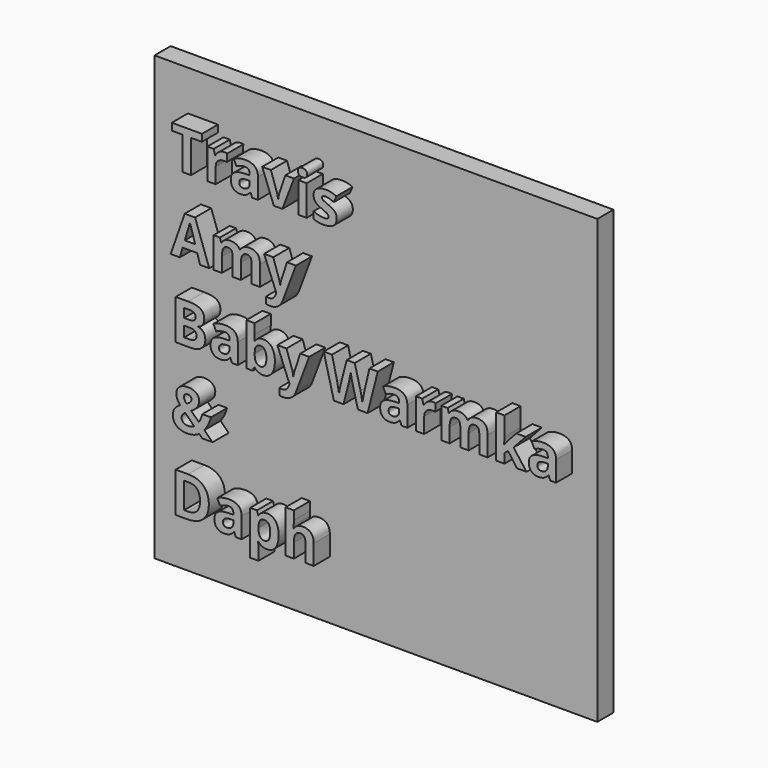
from build123d import *

# Parameters (mm, degrees)
F0_TEXT_SIZE = 17.6388888889
F1_DEPTH     = 12.7
F2_W         = 139.7
F2_H         = 139.7
F3_DEPTH     = 6.35


# Not quite as in the source:
# - Text() gives the source's letters only with a copy of the font that has no kerning and outlines rounded to 1/6400 em; it was checked with that copy


with BuildPart() as f1:
    # F0 (on Front) → F1 (new body)
    with BuildSketch(Plane.XZ):
        with Locations((-21.0479750512, 2.0968852922)):
            Text('Travis', F0_TEXT_SIZE, font='Open Sans', font_style=FontStyle.BOLD, text_align=(TextAlign.LEFT, TextAlign.BOTTOM))
        with Locations((-21.0479750512, -21.8920035967)):
            Text('Amy', F0_TEXT_SIZE, font='Open Sans', font_style=FontStyle.BOLD, text_align=(TextAlign.LEFT, TextAlign.BOTTOM))
        with Locations((-21.0479750512, -45.8808924856)):
            Text('Baby Warmka', F0_TEXT_SIZE, font='Open Sans', font_style=FontStyle.BOLD, text_align=(TextAlign.LEFT, TextAlign.BOTTOM))
        with Locations((-21.0479750512, -69.8697813745)):
            Text('&', F0_TEXT_SIZE, font='Open Sans', font_style=FontStyle.BOLD, text_align=(TextAlign.LEFT, TextAlign.BOTTOM))
        with Locations((-21.0479750512, -93.8586702634)):
            Text('Daph', F0_TEXT_SIZE, font='Open Sans', font_style=FontStyle.BOLD, text_align=(TextAlign.LEFT, TextAlign.BOTTOM))
    extrude(amount=F1_DEPTH)

    # F2 (on Front) → F3 (join)
    with BuildSketch(Plane.XZ):
        with Locations((38.6420249488, -42.460601687)):
            Rectangle(F2_W, F2_H)
    extrude(amount=F3_DEPTH)


solid = f1.part
